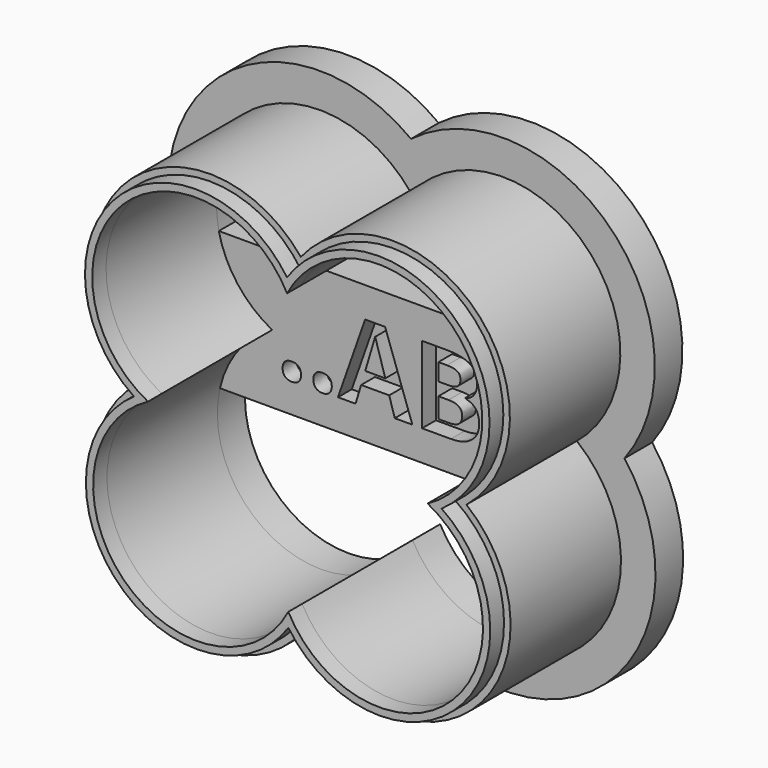
from build123d import *
from build123d import SkipClean  # not in build123d's __all__

# Parameters (mm, degrees)
F1_DEPTH      = 11
F3_DEPTH      = 10
F5_DEPTH      = 10
F7_DEPTH      = 2
F10_DEPTH     = 2
F11_W         = 23.4749444451
F11_H         = 4
F12_DEPTH     = 2
F14_TEXT_SIZE = 6.25
F15_DEPTH     = 1


# Not quite as in the source:
# - after a boolean that leaves OpenCascade's solid faulty, fix() repairs it
# - Text() gives the source's letters only with a copy of the font that has no kerning and outlines rounded to 1/6400 em; it was checked with that copy


with BuildPart() as f1:
    # F0 (on Front) → F1 (new body)
    with BuildSketch(Plane.XZ):
        with BuildLine():
            ThreePointArc((8.9293479726, 0.0340558395), (9.8062955937, 9.879418447), (-0.0311512456, 8.9177315511))
            ThreePointArc((-0.0311512456, 8.9177315511), (-9.8850972107, 9.8005710447), (-8.9057942382, -0.0442561423))
            ThreePointArc((-8.9057942382, -0.0442561423), (-9.7936994074, -9.8918926599), (0.0472553048, -8.9327623639))
            ThreePointArc((0.0472553048, -8.9327623639), (9.8878070421, -9.797839901), (8.9293479726, 0.0340558395))
        make_face()
        with BuildLine():
            ThreePointArc((-8.0911491723, -0.0402078736), (-9.5874784871, 9.5042189943), (-0.0283127003, 8.1051353239))
            ThreePointArc((-0.0283127003, 8.1051353239), (9.509789396, 9.5819534213), (8.1187502981, 0.030964283))
            ThreePointArc((8.1187502981, 0.030964283), (9.5896526998, -9.5020289657), (0.0429703273, -8.1227647296))
            ThreePointArc((0.0429703273, -8.1227647296), (-9.4996553274, -9.5919835604), (-8.0911491723, -0.0402078736))
        make_face(mode=Mode.SUBTRACT)
    extrude(amount=F1_DEPTH)

    # F2 (on Front) → F3 (join)
    with BuildSketch(Plane.XZ):
        with BuildLine():
            ThreePointArc((-0.0333809275, 9.5560272121), (-10.1546317436, 10.0684358843), (-9.545147603, -0.0474333226))
            ThreePointArc((-9.545147603, -0.0474333226), (-10.0603316915, -10.1626498764), (0.0506248229, -9.5697089537))
            ThreePointArc((0.0506248229, -9.5697089537), (10.1576406653, -10.0654027025), (9.566607544, 0.036486298))
            ThreePointArc((9.566607544, 0.036486298), (10.0743082972, 10.1488059131), (-0.0333809275, 9.5560272121))
        make_face()
    extrude(amount=F3_DEPTH)

    # F4 (on face) → F5 (cut)
    with BuildSketch(Plane.XZ.offset(10)):
        with BuildLine():
            ThreePointArc((0.0429703273, -8.1227647296), (9.5896526998, -9.5020289657), (8.1187502981, 0.030964283))
            ThreePointArc((8.1187502981, 0.030964283), (9.509789396, 9.5819534213), (-0.0283127003, 8.1051353239))
            ThreePointArc((-0.0283127003, 8.1051353239), (-9.5874784871, 9.5042189943), (-8.0911491723, -0.0402078736))
            ThreePointArc((-8.0911491723, -0.0402078736), (-9.4996553274, -9.5919835604), (0.0429703273, -8.1227647296))
        make_face()
    with SkipClean():  # cleaning this boolean's faces spoils the solid; the shape is the same uncleaned
        extrude(amount=-F5_DEPTH, mode=Mode.SUBTRACT)

    # F6 (on Front) → F7 (join)
    with BuildSketch(Plane.XZ):
        with BuildLine():
            ThreePointArc((-0.0430466121, 12.3230427318), (-11.5742313321, 11.477243886), (-12.3145134428, -0.0611953123))
            ThreePointArc((-12.3145134428, -0.0611953123), (-11.4659338153, -11.5854281507), (0.0652466307, -12.3336977675))
            ThreePointArc((0.0652466307, -12.3336977675), (11.5781064998, -11.4733363187), (12.3313058534, 0.0470306426))
            ThreePointArc((12.3313058534, 0.0470306426), (11.4839222407, 11.5676051869), (-0.0430466121, 12.3230427318))
        make_face()
    extrude(amount=F7_DEPTH)

    add(f1.part.fix(), mode=Mode.REPLACE)

    # F8 (on face) → F10 (cut)
    with BuildSketch(Plane.XZ.offset(2)):
        with BuildLine():
            ThreePointArc((0.0429703273, -8.1227647296), (9.5896526998, -9.5020289657), (8.1187502981, 0.030964283))
            ThreePointArc((8.1187502981, 0.030964283), (9.509789396, 9.5819534213), (-0.0283127003, 8.1051353239))
            ThreePointArc((-0.0283127003, 8.1051353239), (-9.5874784871, 9.5042189943), (-8.0911491723, -0.0402078736))
            ThreePointArc((-8.0911491723, -0.0402078736), (-9.4996553274, -9.5919835604), (0.0429703273, -8.1227647296))
        make_face()
    extrude(amount=-F10_DEPTH, mode=Mode.SUBTRACT)

    # F11 (on offset) → F12 (join)
    with BuildSketch(Plane.XZ.offset(2)):
        with Locations((-0.1821860569, 2)):
            Rectangle(F11_W, F11_H)
        with Locations((-0.1821860569, -2)):
            Rectangle(F11_W, F11_H)
    extrude(amount=-F12_DEPTH)

    # F14 (on offset) → F15 (cut)
    with BuildSketch(Plane.XZ.offset(2)):
        with Locations((-7.8442382813, -2.2363772828)):
            Text('..AB..', F14_TEXT_SIZE, font='Open Sans', font_style=FontStyle.BOLD, text_align=(TextAlign.LEFT, TextAlign.BOTTOM))
    extrude(amount=-F15_DEPTH, mode=Mode.SUBTRACT)


solid = f1.part
